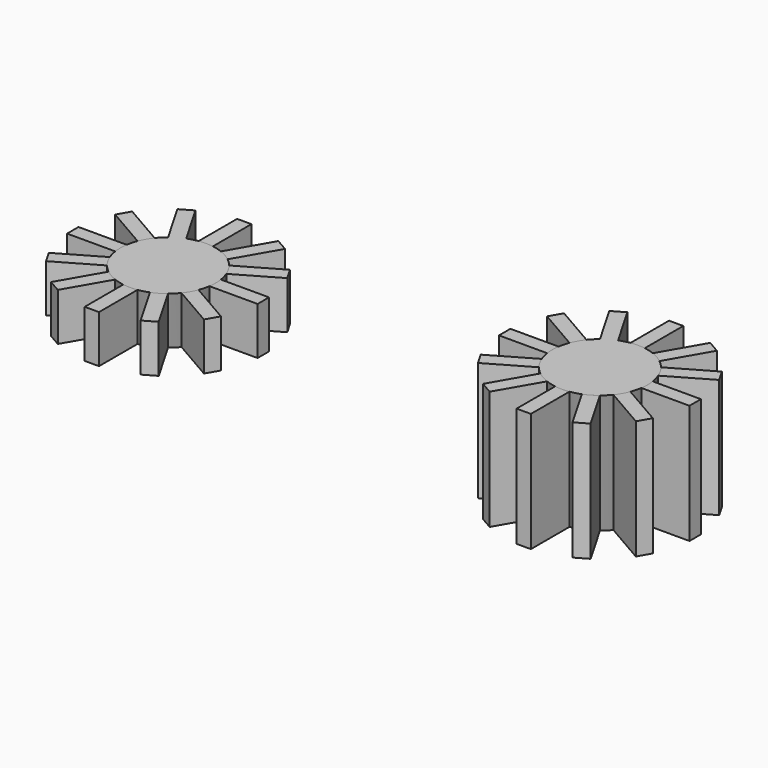
from build123d import *

# Parameters (mm, degrees)
F1_DEPTH = 25
F2_COUNT = 12
F4_DEPTH = 10
F5_COUNT = 12


with BuildPart() as f1:
    # F0 (on Top) → F1 (new body)
    with BuildSketch(Plane.XY):
        with BuildLine():
            ThreePointArc((-1.5, 9.8868599666), (-6.5192024052, -7.5828754441), (10, 0))
            ThreePointArc((10, 0), (7.5828754441, 6.5192024052), (1.5, 9.8868599666))
            ThreePointArc((1.5, 9.8868599666), (0.7521304187, 9.971674876), (0, 10))
            ThreePointArc((0, 10), (-0.7521304187, 9.971674876), (-1.5, 9.8868599666))
        make_face()
        with BuildLine():
            ThreePointArc((0, 10), (0.7521304187, 9.971674876), (1.5, 9.8868599666))
            Line((1.5, 9.8868599666), (1.5, 10))
            Line((1.5, 10), (1.5, 20))
            Line((1.5, 20), (-1.5, 20))
            Line((-1.5, 20), (-1.5, 10))
            Line((-1.5, 10), (-1.5, 9.8868599666))
            ThreePointArc((-1.5, 9.8868599666), (-0.7521304187, 9.971674876), (0, 10))
        make_face()
    extrude(amount=F1_DEPTH)


with BuildPart() as f2_1:
    # F2: instance of F1
    add(f1.part.rotate(Axis((0, 0, 0), (0, 0, -1)), 1 * 360 / F2_COUNT))


with BuildPart() as f2_2:
    # F2: instance of F1
    add(f1.part.rotate(Axis((0, 0, 0), (0, 0, -1)), 2 * 360 / F2_COUNT))


with BuildPart() as f2_3:
    # F2: instance of F1
    add(f1.part.rotate(Axis((0, 0, 0), (0, 0, -1)), 3 * 360 / F2_COUNT))


with BuildPart() as f2_4:
    # F2: instance of F1
    add(f1.part.rotate(Axis((0, 0, 0), (0, 0, -1)), 4 * 360 / F2_COUNT))


with BuildPart() as f2_5:
    # F2: instance of F1
    add(f1.part.rotate(Axis((0, 0, 0), (0, 0, -1)), 5 * 360 / F2_COUNT))


with BuildPart() as f2_6:
    # F2: instance of F1
    add(f1.part.rotate(Axis((0, 0, 0), (0, 0, -1)), 6 * 360 / F2_COUNT))


with BuildPart() as f2_7:
    # F2: instance of F1
    add(f1.part.rotate(Axis((0, 0, 0), (0, 0, -1)), 7 * 360 / F2_COUNT))


with BuildPart() as f2_8:
    # F2: instance of F1
    add(f1.part.rotate(Axis((0, 0, 0), (0, 0, -1)), 8 * 360 / F2_COUNT))


with BuildPart() as f2_9:
    # F2: instance of F1
    add(f1.part.rotate(Axis((0, 0, 0), (0, 0, -1)), 9 * 360 / F2_COUNT))


with BuildPart() as f2_10:
    # F2: instance of F1
    add(f1.part.rotate(Axis((0, 0, 0), (0, 0, -1)), 10 * 360 / F2_COUNT))


with BuildPart() as f2_11:
    # F2: instance of F1
    add(f1.part.rotate(Axis((0, 0, 0), (0, 0, -1)), 11 * 360 / F2_COUNT))


with BuildPart() as f4:
    # F3 (on Top) → F4 (new body)
    with BuildSketch(Plane.XY):
        with BuildLine():
            Line((-94.3747894168, 16.4919358119), (-94.3747894168, 26.4919358119))
            Line((-94.3747894168, 26.4919358119), (-97.3747894168, 26.4919358119))
            Line((-97.3747894168, 26.4919358119), (-97.3747894168, 16.4919358119))
            Line((-97.3747894168, 16.4919358119), (-97.3747894168, 16.3787957786))
            ThreePointArc((-97.3747894168, 16.3787957786), (-95.8747894168, 16.4919358119), (-94.3747894168, 16.3787957786))
            Line((-94.3747894168, 16.3787957786), (-94.3747894168, 16.4919358119))
        make_face()
        with BuildLine():
            ThreePointArc((-85.8747894168, 6.4919358119), (-88.2919139727, 13.0111382171), (-94.3747894168, 16.3787957786))
            ThreePointArc((-94.3747894168, 16.3787957786), (-95.8747894168, 16.4919358119), (-97.3747894168, 16.3787957786))
            ThreePointArc((-97.3747894168, 16.3787957786), (-102.393991822, -1.0909396321), (-85.8747894168, 6.4919358119))
        make_face()
    extrude(amount=F4_DEPTH)


with BuildPart() as f5_1:
    # F5: instance of F4
    add(f4.part.rotate(Axis((-95.8747894168, 6.4919358119, 0), (0, 0, -1)), 1 * 360 / F5_COUNT))


with BuildPart() as f5_2:
    # F5: instance of F4
    add(f4.part.rotate(Axis((-95.8747894168, 6.4919358119, 0), (0, 0, -1)), 2 * 360 / F5_COUNT))


with BuildPart() as f5_3:
    # F5: instance of F4
    add(f4.part.rotate(Axis((-95.8747894168, 6.4919358119, 0), (0, 0, -1)), 3 * 360 / F5_COUNT))


with BuildPart() as f5_4:
    # F5: instance of F4
    add(f4.part.rotate(Axis((-95.8747894168, 6.4919358119, 0), (0, 0, -1)), 4 * 360 / F5_COUNT))


with BuildPart() as f5_5:
    # F5: instance of F4
    add(f4.part.rotate(Axis((-95.8747894168, 6.4919358119, 0), (0, 0, -1)), 5 * 360 / F5_COUNT))


with BuildPart() as f5_6:
    # F5: instance of F4
    add(f4.part.rotate(Axis((-95.8747894168, 6.4919358119, 0), (0, 0, -1)), 6 * 360 / F5_COUNT))


with BuildPart() as f5_7:
    # F5: instance of F4
    add(f4.part.rotate(Axis((-95.8747894168, 6.4919358119, 0), (0, 0, -1)), 7 * 360 / F5_COUNT))


with BuildPart() as f5_8:
    # F5: instance of F4
    add(f4.part.rotate(Axis((-95.8747894168, 6.4919358119, 0), (0, 0, -1)), 8 * 360 / F5_COUNT))


with BuildPart() as f5_9:
    # F5: instance of F4
    add(f4.part.rotate(Axis((-95.8747894168, 6.4919358119, 0), (0, 0, -1)), 9 * 360 / F5_COUNT))


with BuildPart() as f5_10:
    # F5: instance of F4
    add(f4.part.rotate(Axis((-95.8747894168, 6.4919358119, 0), (0, 0, -1)), 10 * 360 / F5_COUNT))


with BuildPart() as f5_11:
    # F5: instance of F4
    add(f4.part.rotate(Axis((-95.8747894168, 6.4919358119, 0), (0, 0, -1)), 11 * 360 / F5_COUNT))


solid = Compound([f1.part, f2_1.part, f2_2.part, f2_3.part, f2_4.part, f2_5.part, f2_6.part, f2_7.part, f2_8.part, f2_9.part, f2_10.part, f2_11.part, f4.part, f5_1.part, f5_2.part, f5_3.part, f5_4.part, f5_5.part, f5_6.part, f5_7.part, f5_8.part, f5_9.part, f5_10.part, f5_11.part])
